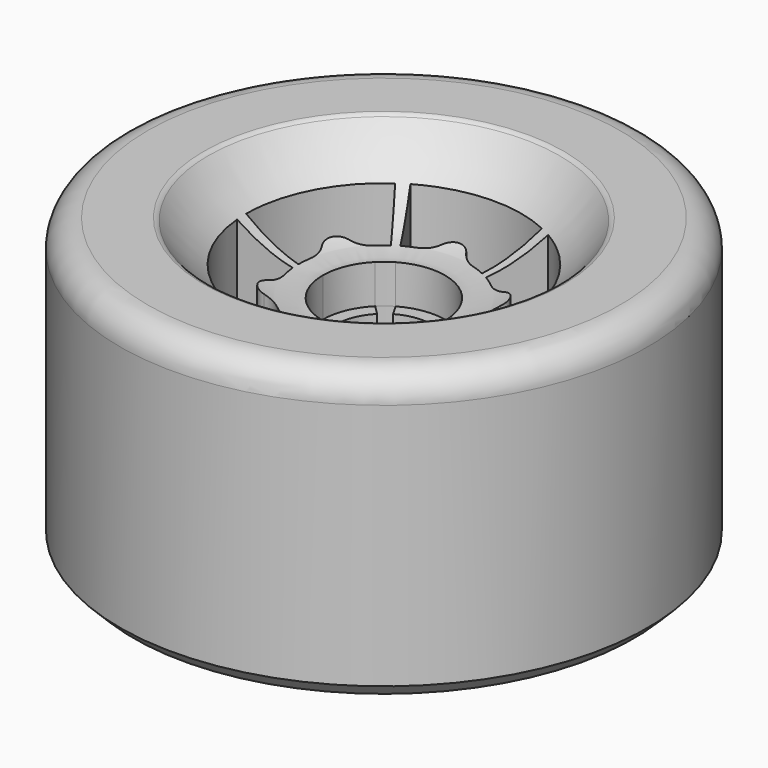
from build123d import *
from build123d import SkipClean  # not in build123d's __all__

# Parameters (mm, degrees)
F2_R     = 5
F3_R     = 1
F5_DEPTH = 137.1
F6_SIZE  = 2.5
F8_START = -17.7
F8_DEPTH = 14.6
F9_DEPTH = 48.5


with BuildPart() as f1:
    # F0 (on Front) → F1 (revolve)
    with BuildSketch(Plane.XZ):
        with BuildLine():
            Line((-4.5753624401, 7.7684287429), (-20.1983146344, 7.7684287429))
            Line((-20.1983146344, 7.7684287429), (-20.1983146344, -18.2315712571))
            Line((-20.1983146344, -18.2315712571), (-20.1983146344, -44.2315712571))
            Line((-20.1983146344, -44.2315712571), (-3.3738550264, -44.2315712571))
            add(Edge.make_bspline(
                [(16.3016853656, -33.5557516078), (-3.3738550264, -33.5557516078), (-3.3738550264, -44.2315712571)],
                knots=[4.7123889804, 4.7123889804, 4.7123889804, 6.2831853072, 6.2831853072, 6.2831853072], degree=2, weights=[1, 0.7071067812, 1]))
            Line((16.3016853656, -33.5557516078), (16.3016853656, -4.9278230367))
            add(Edge.make_bspline(
                [(-4.5753624401, 7.7684287429), (5.471138744, -6.8286280839), (16.3016853656, -4.9278230367)],
                knots=[1.0795611751, 1.0795611751, 1.0795611751, 2.7809467306, 2.7809467306, 2.7809467306], degree=2, weights=[1, 0.6594625172, 1]))
        make_face()
    revolve(axis=Axis((27.3016853656, 0, -31.2315712571), (0, 0, -1)))

    # F2
    f2_edges = [f1.edges().sort_by_distance(p)[0] for p in [
        (74.801685, 0, 7.768429),
    ]]
    fillet(f2_edges, radius=F2_R)

    # F3
    f3_edges = [f1.edges().sort_by_distance(p)[0] for p in [
        (59.178733, 0, 7.768429),
    ]]
    fillet(f3_edges, radius=F3_R)

    # F4 (on face) → F5 (cut)
    with BuildSketch(Plane(origin=(0, 0, -44.2315712571), x_dir=(1, 0, 0), z_dir=(0, 0, -1))):
        with BuildLine():
            Line((34.9946483489, 13.3246027477), (39.6944904862, 21.4649681171))
            ThreePointArc((39.6944904862, 21.4649681171), (28.3828184998, 24.7620198322), (16.8268338493, 22.463391568))
            Line((16.8268338493, 22.463391568), (20.7993120784, 13.9443845142))
            ThreePointArc((20.7993120784, 13.9443845142), (21.9560760046, 14.4274453181), (23.1483254084, 14.8147331704))
            ThreePointArc((23.1483254084, 14.8147331704), (24.7046093894, 15.560315416), (25.9147394877, 16.7905584243))
            ThreePointArc((25.9147394877, 16.7905584243), (28.0818584987, 17.8689025282), (30.1467470863, 16.6057849821))
            ThreePointArc((30.1467470863, 16.6057849821), (31.2450495312, 15.2747536324), (32.7304296074, 14.3963694661))
            ThreePointArc((32.7304296074, 14.3963694661), (33.8843877817, 13.9066439786), (34.9946483489, 13.3246027477))
        make_face()
        with BuildLine():
            Line((19.6087223824, 13.3246027477), (14.9088802451, 21.4649681171))
            ThreePointArc((14.9088802451, 21.4649681171), (6.397713709, 13.3172986752), (2.6103918545, 2.16020827))
            Line((2.6103918545, 2.16020827), (11.9743074926, 1.3409718055))
            ThreePointArc((11.9743074926, 1.3409718055), (12.134346528, 2.5842891537), (12.3950701111, 3.8104513512))
            ThreePointArc((12.3950701111, 3.8104513512), (12.5275189363, 5.531023937), (12.0671622875, 7.1941488482))
            ThreePointArc((12.0671622875, 7.1941488482), (12.216848405, 9.6101010167), (14.3431845816, 10.7667882165))
            ThreePointArc((14.3431845816, 10.7667882165), (16.0450427662, 11.0524303599), (17.5484358066, 11.899615157))
            ThreePointArc((17.5484358066, 11.899615157), (18.5495296068, 12.6541095072), (19.6087223824, 13.3246027477))
        make_face()
        with BuildLine():
            Line((11.9157593991, 0), (2.5160751245, 0))
            ThreePointArc((2.5160751245, 0), (5.3165805748, -11.444721157), (13.0852433707, -20.3031832979))
            Line((13.0852433707, -20.3031832979), (18.4766807798, -12.6034127087))
            ThreePointArc((18.4766807798, -12.6034127087), (17.4799558889, -11.8431561643), (16.5484300683, -11.0042818192))
            ThreePointArc((16.5484300683, -11.0042818192), (15.1245949126, -10.029291479), (13.4541081654, -9.5964095761))
            ThreePointArc((13.4541081654, -9.5964095761), (11.4366752719, -8.2588015114), (11.498122861, -5.8389967656))
            ThreePointArc((11.498122861, -5.8389967656), (12.1016786007, -4.2223232725), (12.1196915649, -2.496754309))
            ThreePointArc((12.1196915649, -2.496754309), (11.9668271907, -1.2525344714), (11.9157593991, 0))
        make_face()
        with BuildLine():
            Line((19.6087223824, -13.3246027477), (14.9088802451, -21.4649681171))
            ThreePointArc((14.9088802451, -21.4649681171), (26.2205522314, -24.7620198322), (37.7765368819, -22.463391568))
            Line((37.7765368819, -22.463391568), (33.8040586528, -13.9443845142))
            ThreePointArc((33.8040586528, -13.9443845142), (32.6472947266, -14.4274453181), (31.4550453228, -14.8147331704))
            ThreePointArc((31.4550453228, -14.8147331704), (29.8987613419, -15.560315416), (28.6886312435, -16.7905584243))
            ThreePointArc((28.6886312435, -16.7905584243), (26.5215122325, -17.8689025282), (24.4566236449, -16.6057849821))
            ThreePointArc((24.4566236449, -16.6057849821), (23.3583212001, -15.2747536324), (21.8729411239, -14.3963694661))
            ThreePointArc((21.8729411239, -14.3963694661), (20.7189829495, -13.9066439786), (19.6087223824, -13.3246027477))
        make_face()
        with BuildLine():
            Line((34.9946483489, -13.3246027477), (39.6944904862, -21.4649681171))
            ThreePointArc((39.6944904862, -21.4649681171), (48.2056570222, -13.3172986752), (51.9929788768, -2.16020827))
            Line((51.9929788768, -2.16020827), (42.6290632387, -1.3409718055))
            ThreePointArc((42.6290632387, -1.3409718055), (42.4690242033, -2.5842891537), (42.2083006201, -3.8104513512))
            ThreePointArc((42.2083006201, -3.8104513512), (42.0758517949, -5.531023937), (42.5362084437, -7.1941488482))
            ThreePointArc((42.5362084437, -7.1941488482), (42.3865223262, -9.6101010167), (40.2601861496, -10.7667882165))
            ThreePointArc((40.2601861496, -10.7667882165), (38.558327965, -11.0524303599), (37.0549349246, -11.899615157))
            ThreePointArc((37.0549349246, -11.899615157), (36.0538411244, -12.6541095072), (34.9946483489, -13.3246027477))
        make_face()
        with BuildLine():
            Line((42.6876113321, 0), (52.0872956067, 0))
            ThreePointArc((52.0872956067, 0), (49.2867901564, 11.444721157), (41.5181273605, 20.3031832979))
            Line((41.5181273605, 20.3031832979), (36.1266899514, 12.6034127087))
            ThreePointArc((36.1266899514, 12.6034127087), (37.1234148423, 11.8431561643), (38.0549406629, 11.0042818192))
            ThreePointArc((38.0549406629, 11.0042818192), (39.4787758187, 10.029291479), (41.1492625658, 9.5964095761))
            ThreePointArc((41.1492625658, 9.5964095761), (43.1666954593, 8.2588015114), (43.1052478703, 5.8389967656))
            ThreePointArc((43.1052478703, 5.8389967656), (42.5016921306, 4.2223232725), (42.4836791664, 2.496754309))
            ThreePointArc((42.4836791664, 2.496754309), (42.6365435405, 1.2525344714), (42.6876113321, 0))
        make_face()
    extrude(amount=-F5_DEPTH, mode=Mode.SUBTRACT)

    # F6
    f6_edges = [f1.edges().sort_by_distance(p)[0] for p in [
        (74.801685, 0, -44.231571),
    ]]
    chamfer(f6_edges, length=F6_SIZE)

    # F7 (on face) → F8 (join)
    with BuildSketch(Plane(origin=(0, 0, -44.2315712571), x_dir=(1, 0, 0), z_dir=(0, 0, -1)).offset(F8_START)):
        with BuildLine():
            Line((35.9378152274, 0), (38.3016853656, 0))
            ThreePointArc((38.3016853656, 0), (33.9980610847, 8.7268867432), (24.4546758695, 10.6251840892))
            Line((24.4546758695, 10.6251840892), (25.0664904814, 8.3418608727))
            ThreePointArc((25.0664904814, 8.3418608727), (32.5590281214, 6.851502473), (35.9378152274, 0))
        make_face()
        with BuildLine():
            ThreePointArc((37.9268694548, -2.8470094961), (38.2075788407, -1.4357881144), (38.3016853656, 0))
            Line((38.3016853656, 0), (35.9378152274, 0))
            ThreePointArc((35.9378152274, 0), (35.8639319392, -1.1272411464), (35.6435462383, -2.2351948842))
            Line((35.6435462383, -2.2351948842), (37.9268694548, -2.8470094961))
        make_face()
        with BuildLine():
            Line((25.0664904814, 8.3418608727), (24.4546758695, 10.6251840892))
            ThreePointArc((24.4546758695, 10.6251840892), (23.0921676096, 10.1626748576), (21.8016853656, 9.5262794416))
            Line((21.8016853656, 9.5262794416), (22.9836204347, 7.4791078507))
            ThreePointArc((22.9836204347, 7.4791078507), (23.9967815478, 7.9787436194), (25.0664904814, 8.3418608727))
        make_face()
        with BuildLine():
            ThreePointArc((21.8016853656, -9.5262794416), (31.5112031216, -10.1626748576), (37.9268694548, -2.8470094961))
            Line((37.9268694548, -2.8470094961), (35.6435462383, -2.2351948842))
            ThreePointArc((35.6435462383, -2.2351948842), (30.6065891835, -7.9787436194), (22.9836204347, -7.4791078507))
            Line((22.9836204347, -7.4791078507), (21.8016853656, -9.5262794416))
        make_face()
        with BuildLine():
            Line((22.9836204347, 7.4791078507), (21.8016853656, 9.5262794416))
            ThreePointArc((21.8016853656, 9.5262794416), (16.3957918905, 1.4357881144), (19.5235107726, -7.7781745931))
            Line((19.5235107726, -7.7781745931), (21.1950193771, -6.1066659885))
            ThreePointArc((21.1950193771, -6.1066659885), (18.739438792, 1.1272411464), (22.9836204347, 7.4791078507))
        make_face()
        with BuildLine():
            ThreePointArc((19.5235107726, -7.7781745931), (20.6053096465, -8.7268867432), (21.8016853656, -9.5262794416))
            Line((21.8016853656, -9.5262794416), (22.9836204347, -7.4791078507))
            ThreePointArc((22.9836204347, -7.4791078507), (22.0443426099, -6.851502473), (21.1950193771, -6.1066659885))
            Line((21.1950193771, -6.1066659885), (19.5235107726, -7.7781745931))
        make_face()
    extrude(amount=-F8_DEPTH)

    # F7 (on face) → F9 (cut)
    with BuildSketch(Plane(origin=(0, 0, -44.2315712571), x_dir=(1, 0, 0), z_dir=(0, 0, -1))):
        with BuildLine():
            Line((25.0664904814, 8.3418608727), (24.4546758695, 10.6251840892))
            ThreePointArc((24.4546758695, 10.6251840892), (23.0921676096, 10.1626748576), (21.8016853656, 9.5262794416))
            Line((21.8016853656, 9.5262794416), (22.9836204347, 7.4791078507))
            ThreePointArc((22.9836204347, 7.4791078507), (23.9967815478, 7.9787436194), (25.0664904814, 8.3418608727))
        make_face()
        with BuildLine():
            ThreePointArc((19.5235107726, -7.7781745931), (20.6053096465, -8.7268867432), (21.8016853656, -9.5262794416))
            Line((21.8016853656, -9.5262794416), (22.9836204347, -7.4791078507))
            ThreePointArc((22.9836204347, -7.4791078507), (22.0443426099, -6.851502473), (21.1950193771, -6.1066659885))
            Line((21.1950193771, -6.1066659885), (19.5235107726, -7.7781745931))
        make_face()
        with BuildLine():
            ThreePointArc((37.9268694548, -2.8470094961), (38.2075788407, -1.4357881144), (38.3016853656, 0))
            Line((38.3016853656, 0), (35.9378152274, 0))
            ThreePointArc((35.9378152274, 0), (35.8639319392, -1.1272411464), (35.6435462383, -2.2351948842))
            Line((35.6435462383, -2.2351948842), (37.9268694548, -2.8470094961))
        make_face()
    with SkipClean():  # cleaning this boolean's faces spoils the solid; the shape is the same uncleaned
        extrude(amount=-F9_DEPTH, mode=Mode.SUBTRACT)


solid = f1.part
